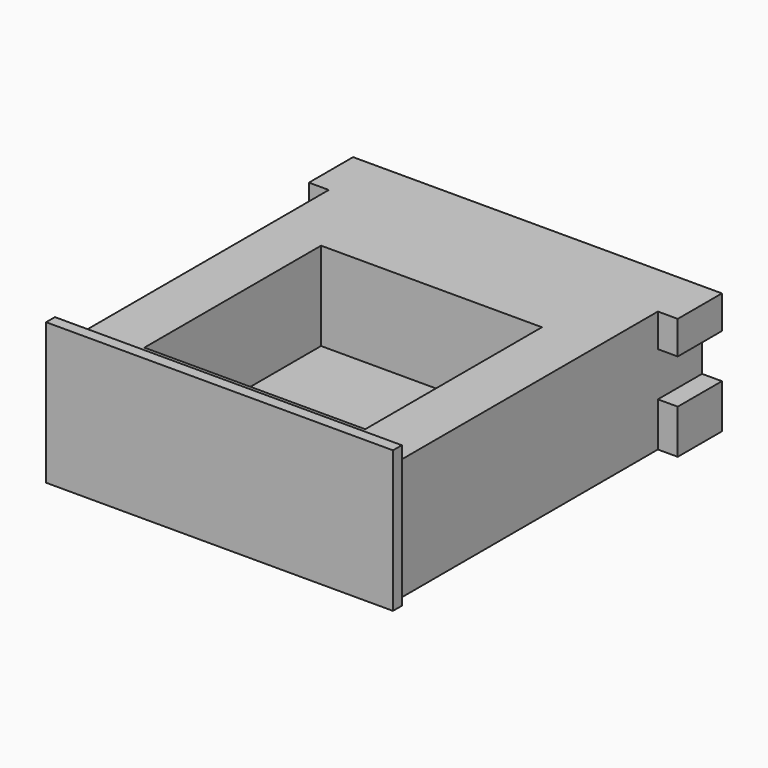
from build123d import *

# Parameters (mm, degrees)
F0_W     = 18.923
F0_H     = 6.985
F1_DEPTH = 22.86
F3_DEPTH = 0.635
F4_W     = 12.7
F4_H     = 12.7
F5_DEPTH = 5.08
F4_W_2   = 1.143
F4_H_2   = 3.175
F6_DEPTH = 6.985
F7_W     = 1.143
F7_H     = 2.54
F8_DEPTH = 12.7


# Not quite as in the source:
# - a feature names something its author has since deleted; it is built from what else it names


with BuildPart() as f1:
    # F0 (on Front) → F1 (new body)
    with BuildSketch(Plane.XZ):
        with Locations((0, -0.3175)):
            Rectangle(F0_W, F0_H)
    extrude(amount=F1_DEPTH)

    # F2 (on face) → F3 (join)
    with BuildSketch(Plane.XZ.offset(22.86)):
        Polygon((9.9764279214, 4.318), (-9.9695, 4.318), (-9.9695, -3.81), (-9.4615, -3.81), (-9.4615, 3.175), (9.4615, 3.175), (9.4615, -3.81), (9.9764279214, -3.81), align=None)
    extrude(amount=-F3_DEPTH)

    # F4 (on face) → F5 (cut)
    with BuildSketch(Plane.XY.offset(3.175)):
        with Locations((0, -13.97)):
            Rectangle(F4_W, F4_H)
    extrude(amount=-F5_DEPTH, mode=Mode.SUBTRACT)

    # F4 (on face) → F6 (join, through all)
    with BuildSketch(Plane.XY.offset(3.175)):
        with Locations((-10.033, -1.5875)):
            Rectangle(F4_W_2, F4_H_2)
        with Locations((10.033, -1.5875)):
            Rectangle(F4_W_2, F4_H_2)
    extrude(amount=-F6_DEPTH)

    # F7 (on face) → F8 (cut)
    with BuildSketch(Plane.XZ):
        with Locations((10.033, 0)):
            Rectangle(F7_W, F7_H)
        with Locations((-10.033, 0)):
            Rectangle(F7_W, F7_H)
    extrude(amount=F8_DEPTH, mode=Mode.SUBTRACT)


solid = f1.part
